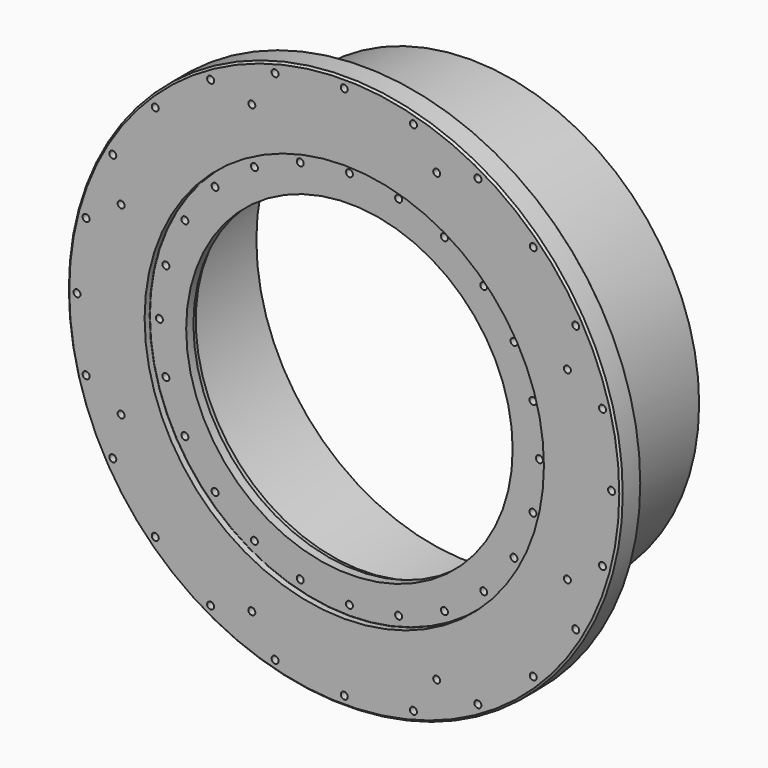
from build123d import *

# Parameters (mm, degrees)
F0_R             = 430
F0_R_2           = 250
F1_DEPTH         = 245
F2_R             = 514.2941305418
F2_R_2           = 430
F2_R_3           = 355
F3_DEPTH         = 205
F4_R             = 332.5
F4_R_2           = 250
F4_R_3           = 222.4010039599
F5_DEPTH         = 210
F6_R             = 310
F6_R_2           = 214.2151850965
F7_DEPTH         = 10
F10_R            = 5.9
F11_DEPTH        = 35
F11_COPIES_COUNT = 24
F12_R            = 5.435
F13_DEPTH        = 100
F14_R            = 5.4
F15_DEPTH        = 331
F16_R            = 5.4
F17_DEPTH        = 50
F18_R            = 3
F19_SIZE         = 3
F20_R            = 4
F21_R            = 0.5


# Not quite as in the source:
# - a pattern or mirror of a feature is missing from the dataset's text; its kind, count and spacing are read off the source's solid


with BuildPart() as f1:
    # F0 (on Front) → F1 (new body)
    with BuildSketch(Plane.XZ):
        Circle(F0_R)
        Circle(F0_R_2, mode=Mode.SUBTRACT)
    extrude(amount=F1_DEPTH)

    # F2 (on face) → F3 (cut)
    with BuildSketch(Plane(origin=(0, 0, 0), x_dir=(-1, 0, 0), z_dir=(0, 1, 0))):
        Circle(F2_R)
        Circle(F2_R_2, mode=Mode.SUBTRACT)
        Circle(F2_R_2)
        Circle(F2_R_3, mode=Mode.SUBTRACT)
    extrude(amount=-F3_DEPTH, mode=Mode.SUBTRACT)

    # F4 (on face) → F5 (cut)
    with BuildSketch(Plane(origin=(0, 0, 0), x_dir=(-1, 0, 0), z_dir=(0, 1, 0))):
        Circle(F4_R)
        Circle(F4_R_2, mode=Mode.SUBTRACT)
        Circle(F4_R_2)
        Circle(F4_R_3, mode=Mode.SUBTRACT)
    extrude(amount=-F5_DEPTH, mode=Mode.SUBTRACT)

    # F6 (on face) → F7 (cut)
    with BuildSketch(Plane.XZ.offset(245)):
        Circle(F6_R)
        Circle(F6_R_2, mode=Mode.SUBTRACT)
    extrude(amount=-F7_DEPTH, mode=Mode.SUBTRACT)

    # F8 (on Top) → F9 (revolve, cut)
    with BuildSketch(Plane.XY):
        with BuildLine():
            ThreePointArc((257.3416655686, -218.687665826), (257.7599514345, -218.3549462248), (257.9471291382, -217.8543167153))
            Line((257.9471291382, -217.8543167153), (259.225389771, -203.243730826))
            Line((259.225389771, -203.243730826), (236.3019734621, -203.243730826))
            Line((236.3019734621, -203.243730826), (252.4756557438, -253.856505284))
            Line((252.4756557438, -253.856505284), (254.25, -220))
            Line((254.25, -220), (257.3416655686, -218.687665826))
        make_face()
    revolve(axis=Axis((0, -156.0075889291, 0), (0, -1, 0)), mode=Mode.SUBTRACT)

    # F10 (on face) → F11 (cut)
    with BuildSketch(Plane(origin=(0, 0, 0), x_dir=(-1, 0, 0), z_dir=(0, 1, 0))):
        with Locations((342.5, 0)):
            Circle(F10_R)
    f11 = extrude(amount=-F11_DEPTH, mode=Mode.SUBTRACT)

    # F11_copies: F11 ×24 about axis
    f11_copies_axis = Axis((0, 0, 0), (0, 1, 0))
    for i in range(1, F11_COPIES_COUNT):
        add(f11.rotate(f11_copies_axis, i * 360 / F11_COPIES_COUNT), mode=Mode.SUBTRACT)

    # F12 (on face) → F13 (cut)
    with BuildSketch(Plane(origin=(0, -205, 0), x_dir=(-1, 0, 0), z_dir=(0, 1, 0))):
        with Locations((0, 415)):
            Circle(F12_R)
        with Locations((-107.4099037175, 400.85921791)):
            Circle(F12_R)
        with Locations((-207.5, 359.4005425705)):
            Circle(F12_R)
        with Locations((-293.4493141924, 293.4493141924)):
            Circle(F12_R)
        with Locations((-359.4005425705, 207.5)):
            Circle(F12_R)
        with Locations((-400.85921791, 107.4099037175)):
            Circle(F12_R)
        with Locations((-415, 0)):
            Circle(F12_R)
        with Locations((-400.85921791, -107.4099037175)):
            Circle(F12_R)
        with Locations((-359.4005425705, -207.5)):
            Circle(F12_R)
        with Locations((-293.4493141924, -293.4493141924)):
            Circle(F12_R)
        with Locations((-207.5, -359.4005425705)):
            Circle(F12_R)
        with Locations((-107.4099037175, -400.85921791)):
            Circle(F12_R)
        with Locations((0, -415)):
            Circle(F12_R)
        with Locations((107.4099037175, -400.85921791)):
            Circle(F12_R)
        with Locations((207.5, -359.4005425705)):
            Circle(F12_R)
        with Locations((293.4493141924, -293.4493141924)):
            Circle(F12_R)
        with Locations((359.4005425705, -207.5)):
            Circle(F12_R)
        with Locations((400.85921791, -107.4099037175)):
            Circle(F12_R)
        with Locations((415, 0)):
            Circle(F12_R)
        with Locations((400.85921791, 107.4099037175)):
            Circle(F12_R)
        with Locations((359.4005425705, 207.5)):
            Circle(F12_R)
        with Locations((293.4493141924, 293.4493141924)):
            Circle(F12_R)
        with Locations((207.5, 359.4005425705)):
            Circle(F12_R)
        with Locations((107.4099037175, 400.85921791)):
            Circle(F12_R)
    extrude(amount=-F13_DEPTH, mode=Mode.SUBTRACT)

    # F14 (on face) → F15 (cut)
    with BuildSketch(Plane(origin=(0, -210, 0), x_dir=(-1, 0, 0), z_dir=(0, 1, 0))):
        with Locations((0, 295)):
            Circle(F14_R)
        with Locations((-76.3516183052, 284.9481187553)):
            Circle(F14_R)
        with Locations((-147.5, 255.4774941164)):
            Circle(F14_R)
        with Locations((-208.59650045, 208.59650045)):
            Circle(F14_R)
        with Locations((-255.4774941164, 147.5)):
            Circle(F14_R)
        with Locations((-284.9481187553, 76.3516183052)):
            Circle(F14_R)
        with Locations((-295, 0)):
            Circle(F14_R)
        with Locations((-284.9481187553, -76.3516183052)):
            Circle(F14_R)
        with Locations((-255.4774941164, -147.5)):
            Circle(F14_R)
        with Locations((-208.59650045, -208.59650045)):
            Circle(F14_R)
        with Locations((-147.5, -255.4774941164)):
            Circle(F14_R)
        with Locations((-76.3516183052, -284.9481187553)):
            Circle(F14_R)
        with Locations((0, -295)):
            Circle(F14_R)
        with Locations((76.3516183052, -284.9481187553)):
            Circle(F14_R)
        with Locations((147.5, -255.4774941164)):
            Circle(F14_R)
        with Locations((208.59650045, -208.59650045)):
            Circle(F14_R)
        with Locations((255.4774941164, -147.5)):
            Circle(F14_R)
        with Locations((284.9481187553, -76.3516183052)):
            Circle(F14_R)
        with Locations((295, 0)):
            Circle(F14_R)
        with Locations((284.9481187553, 76.3516183052)):
            Circle(F14_R)
        with Locations((255.4774941164, 147.5)):
            Circle(F14_R)
        with Locations((208.59650045, 208.59650045)):
            Circle(F14_R)
        with Locations((147.5, 255.4774941164)):
            Circle(F14_R)
        with Locations((76.3516183052, 284.9481187553)):
            Circle(F14_R)
    extrude(amount=-F15_DEPTH, mode=Mode.SUBTRACT)

    # F16 (on face) → F17 (cut)
    with BuildSketch(Plane(origin=(0, -205, 0), x_dir=(-1, 0, 0), z_dir=(0, 1, 0))):
        with Locations((-143.5062871369, 346.4548246917)):
            Circle(F16_R)
        with Locations((-346.4548246917, 143.5062871369)):
            Circle(F16_R)
        with Locations((-346.4548246917, -143.5062871369)):
            Circle(F16_R)
        with Locations((-143.5062871369, -346.4548246917)):
            Circle(F16_R)
        with Locations((143.5062871369, -346.4548246917)):
            Circle(F16_R)
        with Locations((346.4548246917, -143.5062871369)):
            Circle(F16_R)
        with Locations((346.4548246917, 143.5062871369)):
            Circle(F16_R)
        with Locations((143.5062871369, 346.4548246917)):
            Circle(F16_R)
    extrude(amount=-F17_DEPTH, mode=Mode.SUBTRACT)

    # F18
    f18_edges = [f1.edges().sort_by_distance(p)[0] for p in [
        (332.5, -210, 0),
    ]]
    fillet(f18_edges, radius=F18_R)

    # F19
    f19_edges = [f1.edges().sort_by_distance(p)[0] for p in [
        (-430, -245, 0),
        (-430, -205, 0),
    ]]
    chamfer(f19_edges, length=F19_SIZE)

    # F20
    f20_edges = [f1.edges().sort_by_distance(p)[0] for p in [
        (355, -205, 0),
    ]]
    fillet(f20_edges, radius=F20_R)

    # F21
    f21_edges = [f1.edges().sort_by_distance(p)[0] for p in [
        (-310, -235, 0),
    ]]
    fillet(f21_edges, radius=F21_R)


solid = f1.part
